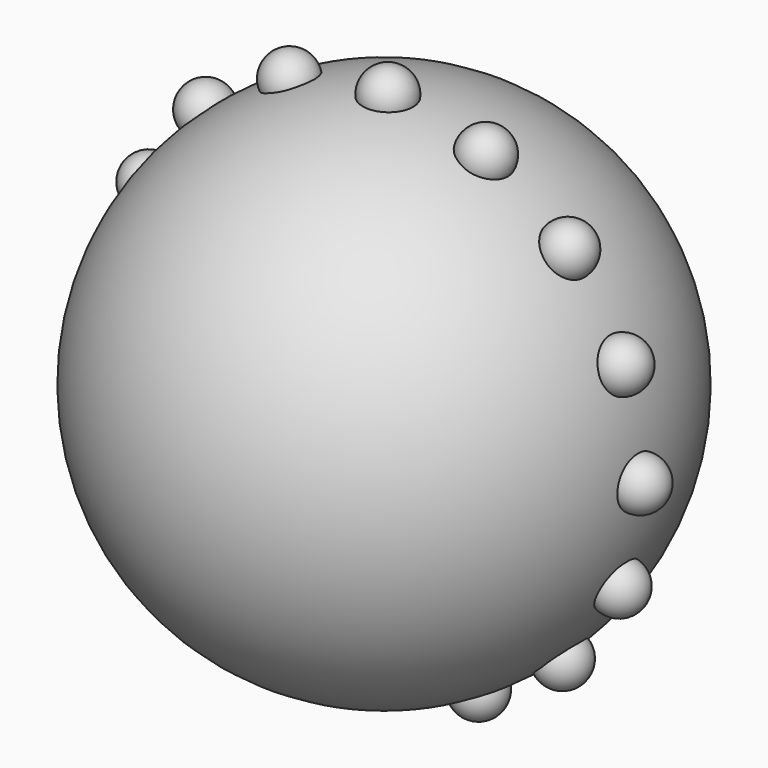
from build123d import *

# Parameters (mm, degrees)
F5_COUNT = 16


# Not quite as in the source:
# - a feature names something its author has since deleted; it is built from what else it names


with BuildPart() as f1:
    # F0 (on Front) → F1 (revolve)
    with BuildSketch(Plane.XZ):
        with BuildLine():
            Line((0, -50), (0, 50))
            ThreePointArc((0, 50), (-50, 0), (0, -50))
        make_face()
    revolve(axis=Axis((0, 0, 5.3528230637), (0, 0, -1)))


with BuildPart() as f3:
    # F2 (on Front) → F3 (revolve)
    with BuildSketch(Plane.XZ):
        with BuildLine():
            ThreePointArc((-41.0540491207, 19.8859551657), (-45.0380591623, 24.781643514), (-50.6411548825, 21.8755432464))
            Line((-50.6411548825, 21.8755432464), (-41.466943359, 17.896367085))
            ThreePointArc((-41.466943359, 17.896367085), (-41.1583607724, 18.8699652072), (-41.0540491207, 19.8859551657))
        make_face()
    revolve(axis=Axis((-46.0540491207, 0, 19.8859551657), (0.9174211523, 0, -0.3979176161)))


with BuildPart() as f5_1:
    # F5: instance of F3
    add(f3.part.rotate(Axis((0, 0.0924132764, 0), (0, -1, 0)), 1 * 360 / F5_COUNT))


with BuildPart() as f5_2:
    # F5: instance of F3
    add(f3.part.rotate(Axis((0, 0.0924132764, 0), (0, -1, 0)), 2 * 360 / F5_COUNT))


with BuildPart() as f5_3:
    # F5: instance of F3
    add(f3.part.rotate(Axis((0, 0.0924132764, 0), (0, -1, 0)), 3 * 360 / F5_COUNT))


with BuildPart() as f5_4:
    # F5: instance of F3
    add(f3.part.rotate(Axis((0, 0.0924132764, 0), (0, -1, 0)), 4 * 360 / F5_COUNT))


with BuildPart() as f5_5:
    # F5: instance of F3
    add(f3.part.rotate(Axis((0, 0.0924132764, 0), (0, -1, 0)), 5 * 360 / F5_COUNT))


with BuildPart() as f5_6:
    # F5: instance of F3
    add(f3.part.rotate(Axis((0, 0.0924132764, 0), (0, -1, 0)), 6 * 360 / F5_COUNT))


with BuildPart() as f5_7:
    # F5: instance of F3
    add(f3.part.rotate(Axis((0, 0.0924132764, 0), (0, -1, 0)), 7 * 360 / F5_COUNT))


with BuildPart() as f5_8:
    # F5: instance of F3
    add(f3.part.rotate(Axis((0, 0.0924132764, 0), (0, -1, 0)), 8 * 360 / F5_COUNT))


with BuildPart() as f5_9:
    # F5: instance of F3
    add(f3.part.rotate(Axis((0, 0.0924132764, 0), (0, -1, 0)), 9 * 360 / F5_COUNT))


with BuildPart() as f5_10:
    # F5: instance of F3
    add(f3.part.rotate(Axis((0, 0.0924132764, 0), (0, -1, 0)), 10 * 360 / F5_COUNT))


with BuildPart() as f5_11:
    # F5: instance of F3
    add(f3.part.rotate(Axis((0, 0.0924132764, 0), (0, -1, 0)), 11 * 360 / F5_COUNT))


with BuildPart() as f5_12:
    # F5: instance of F3
    add(f3.part.rotate(Axis((0, 0.0924132764, 0), (0, -1, 0)), 12 * 360 / F5_COUNT))


with BuildPart() as f5_13:
    # F5: instance of F3
    add(f3.part.rotate(Axis((0, 0.0924132764, 0), (0, -1, 0)), 13 * 360 / F5_COUNT))


with BuildPart() as f5_14:
    # F5: instance of F3
    add(f3.part.rotate(Axis((0, 0.0924132764, 0), (0, -1, 0)), 14 * 360 / F5_COUNT))


with BuildPart() as f5_15:
    # F5: instance of F3
    add(f3.part.rotate(Axis((0, 0.0924132764, 0), (0, -1, 0)), 15 * 360 / F5_COUNT))


solid = Compound([f1.part, f3.part, f5_1.part, f5_2.part, f5_3.part, f5_4.part, f5_5.part, f5_6.part, f5_7.part, f5_8.part, f5_9.part, f5_10.part, f5_11.part, f5_12.part, f5_13.part, f5_14.part, f5_15.part])
